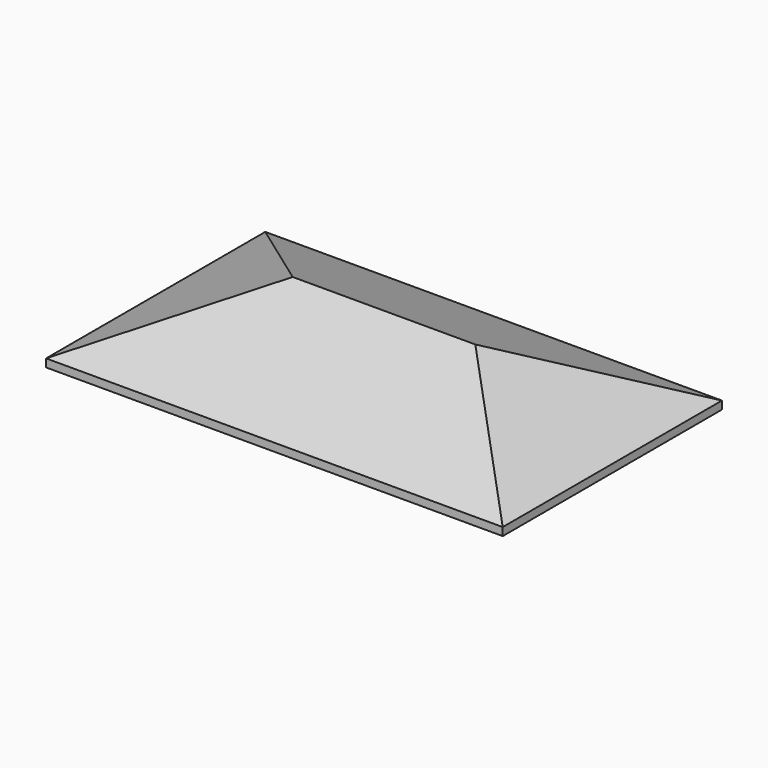
from build123d import *

# Parameters (mm, degrees)
F0_W     = 50.8
F0_H     = 30.48
F1_DEPTH = 7.62
F2_SIZE2 = 6.73099
F2_SIZE  = 15.23999


# Not quite as in the source:
# - a fillet or chamfer is up to 0.001 mm smaller than in the source, because OpenCascade refuses the exact size


with BuildPart() as f1:
    # F0 (on Top) → F1 (new body)
    with BuildSketch(Plane.XY):
        Rectangle(F0_W, F0_H)
    extrude(amount=F1_DEPTH)

    # F2 (size 15.24 and 6.731 in the source; OpenCascade refuses exactly that, so slightly less here)
    f2_edges = [f1.edges().sort_by_distance(p)[0] for p in [
        (-25.4, 0, 7.62),
        (0, 15.24, 7.62),
        (0, -15.24, 7.62),
        (25.4, 0, 7.62),
    ]]
    f2_side = f1.faces().sort_by_distance((0, 0, 7.62))[0]
    chamfer(f2_edges, length=F2_SIZE, length2=F2_SIZE2, reference=f2_side)


solid = f1.part
